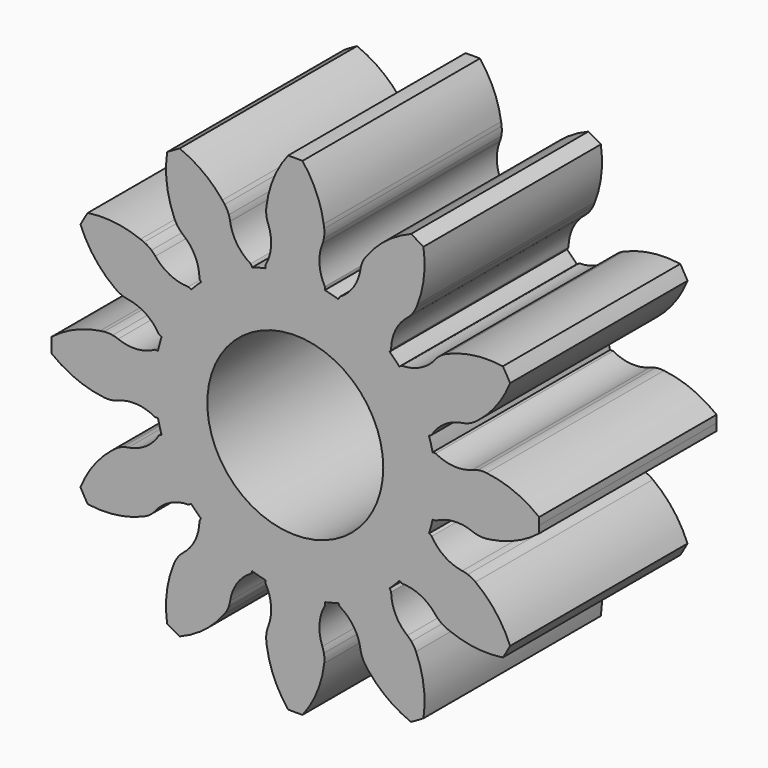
from build123d import *

# Parameters (mm, degrees)
F0_R     = 5.95
F1_DEPTH = 15


with BuildPart() as f1:
    # F0 (on Front) → F1 (new body)
    with BuildSketch(Plane.XZ):
        with BuildLine():
            ThreePointArc((16.4927779447, -0.4881348847), (16.4981943874, -0.2440941538), (16.5, 0))
            ThreePointArc((16.5, 0), (16.4981943874, 0.2440941538), (16.4927779447, 0.4881348847))
            ThreePointArc((16.4927779448, 0.4881348847), (14.8199031267, 1.4716268374), (12.9411319368, 1.9574101163))
            ThreePointArc((12.9411319368, 1.9574101163), (12.6443205895, 1.9691300904), (12.3490470013, 1.936759706))
            ThreePointArc((12.3490470013, 1.936759706), (12.4622046107, 0.9713167566), (12.5, 0))
            ThreePointArc((12.5, 0), (12.4622046107, -0.9713167566), (12.3490470013, -1.936759706))
            ThreePointArc((12.3490470013, -1.936759706), (12.6443205895, -1.9691300904), (12.9411319368, -1.9574101163))
            ThreePointArc((12.9411319368, -1.9574101163), (13.0706718945, -1.9413788034), (13.1998899951, -1.9229319577))
            ThreePointArc((13.1998899951, -1.9229319577), (14.9400467825, -1.4206061985), (16.4927779447, -0.4881348847))
        make_face()
        with BuildLine():
            ThreePointArc((12.3929060418, 4.9346370725), (13.6487631466, 6.2397423346), (14.5272321215, 7.8236517617))
            ThreePointArc((14.5272321215, 7.8236517617), (14.2894191624, 8.25), (14.0390972368, 8.669126183))
            ThreePointArc((14.0390972368, 8.669126183), (12.0985991706, 8.6844177894), (10.2286439528, 8.1657328548))
            ThreePointArc((10.2286439528, 8.1657328548), (9.9657377989, 8.0274769764), (9.7262085627, 7.8518066071))
            ThreePointArc((9.7262085627, 7.8518066071), (10.8253175473, 6.25), (11.6629682687, 4.4972403942))
            ThreePointArc((11.6629682687, 4.4972403942), (11.9348678893, 4.6168436131), (12.1860540692, 4.775399082))
            ThreePointArc((12.1860540692, 4.775399082), (12.2902233069, 4.8540525851), (12.3929060418, 4.9346370725))
        make_face()
        with BuildLine():
            ThreePointArc((14.0390972368, -8.669126183), (14.2894191624, -8.25), (14.5272321215, -7.8236517617))
            ThreePointArc((14.5272321215, -7.8236517617), (13.570226008, -6.1354853373), (12.1860540692, -4.775399082))
            ThreePointArc((12.1860540692, -4.775399082), (11.9348678893, -4.6168436131), (11.6629682687, -4.4972403942))
            ThreePointArc((11.6629682687, -4.4972403942), (10.8253175473, -6.25), (9.7262085627, -7.8518066071))
            ThreePointArc((9.7262085627, -7.8518066071), (9.9657377989, -8.0274769764), (10.2286439528, -8.1657328548))
            ThreePointArc((10.2286439528, -8.1657328548), (10.3488445035, -8.2166193094), (10.4699740841, -8.2652529226))
            ThreePointArc((10.4699740841, -8.2652529226), (12.2281569481, -8.7003044479), (14.0390972368, -8.669126183))
        make_face()
        with BuildLine():
            ThreePointArc((12.5, 0), (12.4622046107, 0.9713167566), (12.3490470013, 1.936759706))
            ThreePointArc((12.3490470013, 1.936759706), (12.163920368, 1.8932016239), (11.9837680157, 1.8322565103))
            ThreePointArc((11.9837680157, 1.8322565103), (10.7230754287, 1.6376307269), (9.5, 2))
            ThreePointArc((9.5, 2), (9.3935439053, 2.0073586069), (9.2870878105, 2))
            ThreePointArc((9.2870878105, 2), (9.4466219941, 1.0056504861), (9.5, 0))
            ThreePointArc((9.5, 0), (9.4466219941, -1.0056504861), (9.2870878105, -2))
            ThreePointArc((9.2870878105, -2), (9.3935439053, -2.0073586069), (9.5, -2))
            ThreePointArc((9.5, -2), (10.7230754287, -1.6376307269), (11.9837680157, -1.8322565103))
            ThreePointArc((11.9837680157, -1.8322565103), (12.163920368, -1.8932016239), (12.3490470013, -1.936759706))
            ThreePointArc((12.3490470013, -1.936759706), (12.4622046107, -0.9713167566), (12.5, 0))
        make_face()
        with BuildLine():
            ThreePointArc((8.2652529226, 10.4699740841), (8.7003044479, 12.2281569481), (8.669126183, 14.0390972368))
            ThreePointArc((8.669126183, 14.0390972368), (8.25, 14.2894191624), (7.8236517617, 14.5272321215))
            ThreePointArc((7.8236517617, 14.5272321215), (6.1354853373, 13.570226008), (4.775399082, 12.1860540692))
            ThreePointArc((4.775399082, 12.1860540692), (4.6168436131, 11.9348678893), (4.4972403942, 11.6629682687))
            ThreePointArc((4.4972403942, 11.6629682687), (6.25, 10.8253175473), (7.8518066071, 9.7262085627))
            ThreePointArc((7.8518066071, 9.7262085627), (8.0274769764, 9.9657377989), (8.1657328548, 10.2286439528))
            ThreePointArc((8.1657328548, 10.2286439528), (8.2166193094, 10.3488445035), (8.2652529226, 10.4699740841))
        make_face()
        with BuildLine():
            ThreePointArc((7.8236517617, -14.5272321215), (8.25, -14.2894191624), (8.669126183, -14.0390972368))
            ThreePointArc((8.669126183, -14.0390972368), (8.6844177894, -12.0985991706), (8.1657328548, -10.2286439528))
            ThreePointArc((8.1657328548, -10.2286439528), (8.0274769764, -9.9657377989), (7.8518066071, -9.7262085627))
            ThreePointArc((7.8518066071, -9.7262085627), (6.25, -10.8253175473), (4.4972403942, -11.6629682687))
            ThreePointArc((4.4972403942, -11.6629682687), (4.6168436131, -11.9348678893), (4.775399082, -12.1860540692))
            ThreePointArc((4.775399082, -12.1860540692), (4.8540525851, -12.2902233069), (4.9346370725, -12.3929060418))
            ThreePointArc((4.9346370725, -12.3929060418), (6.2397423346, -13.6487631466), (7.8236517617, -14.5272321215))
        make_face()
        with BuildLine():
            ThreePointArc((9.7262085627, -7.8518066071), (10.8253175473, -6.25), (11.6629682687, -4.4972403942))
            ThreePointArc((11.6629682687, -4.4972403942), (11.4808648602, -4.4423994832), (11.2943757898, -4.4051033237))
            ThreePointArc((11.2943757898, -4.4051033237), (10.1052710914, -3.9433079029), (9.227241336, -3.0179491924))
            ThreePointArc((9.227241336, -3.0179491924), (9.138726957, -2.9583484045), (9.0428539711, -2.9114930977))
            ThreePointArc((9.0428539711, -2.9114930977), (8.227241336, -4.75), (7.0428539711, -6.3755947128))
            ThreePointArc((7.0428539711, -6.3755947128), (7.13136835, -6.4351955007), (7.227241336, -6.4820508076))
            ThreePointArc((7.227241336, -6.4820508076), (8.4676403645, -6.7797675259), (9.4621192795, -7.578664692))
            ThreePointArc((9.4621192795, -7.578664692), (9.5876632363, -7.7215208848), (9.7262085627, -7.8518066071))
        make_face()
        with BuildLine():
            ThreePointArc((11.6629682687, 4.4972403942), (10.8253175473, 6.25), (9.7262085627, 7.8518066071))
            ThreePointArc((9.7262085627, 7.8518066071), (9.5876632363, 7.7215208848), (9.4621192795, 7.578664692))
            ThreePointArc((9.4621192795, 7.578664692), (8.4676403645, 6.7797675259), (7.227241336, 6.4820508076))
            ThreePointArc((7.227241336, 6.4820508076), (7.13136835, 6.4351955007), (7.0428539711, 6.3755947128))
            ThreePointArc((7.0428539711, 6.3755947128), (8.227241336, 4.75), (9.0428539711, 2.9114930977))
            ThreePointArc((9.0428539711, 2.9114930977), (9.138726957, 2.9583484045), (9.227241336, 3.0179491924))
            ThreePointArc((9.227241336, 3.0179491924), (10.1052710914, 3.9433079029), (11.2943757898, 4.4051033237))
            ThreePointArc((11.2943757898, 4.4051033237), (11.4808648602, 4.4423994832), (11.6629682687, 4.4972403942))
        make_face()
        with BuildLine():
            ThreePointArc((9.5, 0), (9.4466219941, 1.0056504861), (9.2870878105, 2))
            ThreePointArc((9.2870878105, 2), (9.1762953497, 2.4587809285), (9.0428539711, 2.9114930977))
            ThreePointArc((9.0428539711, 2.9114930977), (8.227241336, 4.75), (7.0428539711, 6.3755947128))
            ThreePointArc((7.0428539711, 6.3755947128), (6.7175144213, 6.7175144213), (6.3755947128, 7.0428539711))
            ThreePointArc((6.3755947128, 7.0428539711), (4.75, 8.227241336), (2.9114930977, 9.0428539711))
            ThreePointArc((2.9114930977, 9.0428539711), (2.4587809285, 9.1762953497), (2, 9.2870878105))
            ThreePointArc((2, 9.2870878105), (0, 9.5), (-2, 9.2870878105))
            ThreePointArc((-2, 9.2870878105), (-2.4587809285, 9.1762953497), (-2.9114930977, 9.0428539711))
            ThreePointArc((-2.9114930977, 9.0428539711), (-4.75, 8.227241336), (-6.3755947128, 7.0428539711))
            ThreePointArc((-6.3755947128, 7.0428539711), (-6.7175144213, 6.7175144213), (-7.0428539711, 6.3755947128))
            ThreePointArc((-7.0428539711, 6.3755947128), (-8.227241336, 4.75), (-9.0428539711, 2.9114930977))
            ThreePointArc((-9.0428539711, 2.9114930977), (-9.1762953497, 2.4587809285), (-9.2870878105, 2))
            ThreePointArc((-9.2870878105, 2), (-9.5, 0), (-9.2870878105, -2))
            ThreePointArc((-9.2870878105, -2), (-9.1762953497, -2.4587809285), (-9.0428539711, -2.9114930977))
            ThreePointArc((-9.0428539711, -2.9114930977), (-8.227241336, -4.75), (-7.0428539711, -6.3755947128))
            ThreePointArc((-7.0428539711, -6.3755947128), (-6.7175144213, -6.7175144213), (-6.3755947128, -7.0428539711))
            ThreePointArc((-6.3755947128, -7.0428539711), (-4.75, -8.227241336), (-2.9114930977, -9.0428539711))
            ThreePointArc((-2.9114930977, -9.0428539711), (-2.4587809285, -9.1762953497), (-2, -9.2870878105))
            ThreePointArc((-2, -9.2870878105), (0, -9.5), (2, -9.2870878105))
            ThreePointArc((2, -9.2870878105), (2.4587809285, -9.1762953497), (2.9114930977, -9.0428539711))
            ThreePointArc((2.9114930977, -9.0428539711), (4.75, -8.227241336), (6.3755947128, -7.0428539711))
            ThreePointArc((6.3755947128, -7.0428539711), (6.7175144213, -6.7175144213), (7.0428539711, -6.3755947128))
            ThreePointArc((7.0428539711, -6.3755947128), (8.227241336, -4.75), (9.0428539711, -2.9114930977))
            ThreePointArc((9.0428539711, -2.9114930977), (9.1762953497, -2.4587809285), (9.2870878105, -2))
            ThreePointArc((9.2870878105, -2), (9.4466219941, -1.0056504861), (9.5, 0))
        make_face()
        Circle(F0_R, mode=Mode.SUBTRACT)
        with BuildLine():
            ThreePointArc((-0.4881348847, -16.4927779447), (0, -16.5), (0.4881348847, -16.4927779447))
            ThreePointArc((0.4881348847, -16.4927779448), (1.4716268374, -14.8199031267), (1.9574101163, -12.9411319368))
            ThreePointArc((1.9574101163, -12.9411319368), (1.9691300904, -12.6443205895), (1.936759706, -12.3490470013))
            ThreePointArc((1.936759706, -12.3490470013), (0, -12.5), (-1.936759706, -12.3490470013))
            ThreePointArc((-1.936759706, -12.3490470013), (-1.9691300904, -12.6443205895), (-1.9574101163, -12.9411319368))
            ThreePointArc((-1.9574101163, -12.9411319368), (-1.9413788034, -13.0706718945), (-1.9229319577, -13.1998899951))
            ThreePointArc((-1.9229319577, -13.1998899951), (-1.4206061985, -14.9400467825), (-0.4881348847, -16.4927779447))
        make_face()
        with BuildLine():
            ThreePointArc((4.4972403942, -11.6629682687), (6.25, -10.8253175473), (7.8518066071, -9.7262085627))
            ThreePointArc((7.8518066071, -9.7262085627), (7.7215208848, -9.5876632363), (7.578664692, -9.4621192795))
            ThreePointArc((7.578664692, -9.4621192795), (6.7797675259, -8.4676403645), (6.4820508076, -7.227241336))
            ThreePointArc((6.4820508076, -7.227241336), (6.4351955007, -7.13136835), (6.3755947128, -7.0428539711))
            ThreePointArc((6.3755947128, -7.0428539711), (4.75, -8.227241336), (2.9114930977, -9.0428539711))
            ThreePointArc((2.9114930977, -9.0428539711), (2.9583484045, -9.138726957), (3.0179491924, -9.227241336))
            ThreePointArc((3.0179491924, -9.227241336), (3.9433079029, -10.1052710914), (4.4051033237, -11.2943757898))
            ThreePointArc((4.4051033237, -11.2943757898), (4.4423994832, -11.4808648602), (4.4972403942, -11.6629682687))
        make_face()
        with BuildLine():
            ThreePointArc((7.8518066071, 9.7262085627), (6.25, 10.8253175473), (4.4972403942, 11.6629682687))
            ThreePointArc((4.4972403942, 11.6629682687), (4.4423994832, 11.4808648602), (4.4051033237, 11.2943757898))
            ThreePointArc((4.4051033237, 11.2943757898), (3.9433079029, 10.1052710914), (3.0179491924, 9.227241336))
            ThreePointArc((3.0179491924, 9.227241336), (2.9583484045, 9.138726957), (2.9114930977, 9.0428539711))
            ThreePointArc((2.9114930977, 9.0428539711), (4.75, 8.227241336), (6.3755947128, 7.0428539711))
            ThreePointArc((6.3755947128, 7.0428539711), (6.4351955007, 7.13136835), (6.4820508076, 7.227241336))
            ThreePointArc((6.4820508076, 7.227241336), (6.7797675259, 8.4676403645), (7.578664692, 9.4621192795))
            ThreePointArc((7.578664692, 9.4621192795), (7.7215208848, 9.5876632363), (7.8518066071, 9.7262085627))
        make_face()
        with BuildLine():
            ThreePointArc((1.9229319577, 13.1998899951), (1.4206061985, 14.9400467825), (0.4881348847, 16.4927779447))
            ThreePointArc((0.4881348847, 16.4927779447), (0, 16.5), (-0.4881348847, 16.4927779447))
            ThreePointArc((-0.4881348847, 16.4927779448), (-1.4716268374, 14.8199031267), (-1.9574101163, 12.9411319368))
            ThreePointArc((-1.9574101163, 12.9411319368), (-1.9691300904, 12.6443205895), (-1.936759706, 12.3490470013))
            ThreePointArc((-1.936759706, 12.3490470013), (-0.9713167566, 12.4622046107), (0, 12.5))
            Line((0, 12.5), (1.9229319577, 13.1998899951))
        make_face()
        with BuildLine():
            ThreePointArc((-8.669126183, -14.0390972368), (-8.25, -14.2894191624), (-7.8236517617, -14.5272321215))
            ThreePointArc((-7.8236517617, -14.5272321215), (-6.1354853373, -13.570226008), (-4.775399082, -12.1860540692))
            ThreePointArc((-4.775399082, -12.1860540692), (-4.6168436131, -11.9348678893), (-4.4972403942, -11.6629682687))
            ThreePointArc((-4.4972403942, -11.6629682687), (-6.25, -10.8253175473), (-7.8518066071, -9.7262085627))
            ThreePointArc((-7.8518066071, -9.7262085627), (-8.0274769764, -9.9657377989), (-8.1657328548, -10.2286439528))
            ThreePointArc((-8.1657328548, -10.2286439528), (-8.2166193094, -10.3488445035), (-8.2652529226, -10.4699740841))
            ThreePointArc((-8.2652529226, -10.4699740841), (-8.7003044479, -12.2281569481), (-8.669126183, -14.0390972368))
        make_face()
        with BuildLine():
            ThreePointArc((-1.936759706, -12.3490470013), (0, -12.5), (1.936759706, -12.3490470013))
            ThreePointArc((1.936759706, -12.3490470013), (1.8932016239, -12.163920368), (1.8322565103, -11.9837680157))
            ThreePointArc((1.8322565103, -11.9837680157), (1.6376307269, -10.7230754287), (2, -9.5))
            ThreePointArc((2, -9.5), (2.0073586069, -9.3935439053), (2, -9.2870878105))
            ThreePointArc((2, -9.2870878105), (0, -9.5), (-2, -9.2870878105))
            ThreePointArc((-2, -9.2870878105), (-2.0073586069, -9.3935439053), (-2, -9.5))
            ThreePointArc((-2, -9.5), (-1.6376307269, -10.7230754287), (-1.8322565103, -11.9837680157))
            ThreePointArc((-1.8322565103, -11.9837680157), (-1.8932016239, -12.163920368), (-1.936759706, -12.3490470013))
        make_face()
        with BuildLine():
            ThreePointArc((1.9574101163, 12.9411319368), (1.9413788034, 13.0706718945), (1.9229319577, 13.1998899951))
            Line((1.9229319577, 13.1998899951), (0, 12.5))
            ThreePointArc((0, 12.5), (0.9713167566, 12.4622046107), (1.936759706, 12.3490470013))
            ThreePointArc((1.936759706, 12.3490470013), (1.9691300904, 12.6443205895), (1.9574101163, 12.9411319368))
        make_face()
        with BuildLine():
            ThreePointArc((2, 9.2870878105), (2.0073586069, 9.3935439053), (2, 9.5))
            ThreePointArc((2, 9.5), (1.6376307269, 10.7230754287), (1.8322565103, 11.9837680157))
            ThreePointArc((1.8322565103, 11.9837680157), (1.8932016239, 12.163920368), (1.936759706, 12.3490470013))
            ThreePointArc((1.936759706, 12.3490470013), (0.9713167566, 12.4622046107), (0, 12.5))
            ThreePointArc((0, 12.5), (-0.9713167566, 12.4622046107), (-1.936759706, 12.3490470013))
            ThreePointArc((-1.936759706, 12.3490470013), (-1.8932016239, 12.163920368), (-1.8322565103, 11.9837680157))
            ThreePointArc((-1.8322565103, 11.9837680157), (-1.6376307269, 10.7230754287), (-2, 9.5))
            ThreePointArc((-2, 9.5), (-2.0073586069, 9.3935439053), (-2, 9.2870878105))
            ThreePointArc((-2, 9.2870878105), (0, 9.5), (2, 9.2870878105))
        make_face()
        with BuildLine():
            ThreePointArc((-14.5272321215, -7.8236517617), (-14.2894191624, -8.25), (-14.0390972368, -8.669126183))
            ThreePointArc((-14.0390972368, -8.669126183), (-12.0985991706, -8.6844177894), (-10.2286439528, -8.1657328548))
            ThreePointArc((-10.2286439528, -8.1657328548), (-9.9657377989, -8.0274769764), (-9.7262085627, -7.8518066071))
            ThreePointArc((-9.7262085627, -7.8518066071), (-10.8253175473, -6.25), (-11.6629682687, -4.4972403942))
            ThreePointArc((-11.6629682687, -4.4972403942), (-11.9348678893, -4.6168436131), (-12.1860540692, -4.775399082))
            ThreePointArc((-12.1860540692, -4.775399082), (-12.2902233069, -4.8540525851), (-12.3929060418, -4.9346370725))
            ThreePointArc((-12.3929060418, -4.9346370725), (-13.6487631466, -6.2397423346), (-14.5272321215, -7.8236517617))
        make_face()
        with BuildLine():
            ThreePointArc((-7.8518066071, -9.7262085627), (-6.25, -10.8253175473), (-4.4972403942, -11.6629682687))
            ThreePointArc((-4.4972403942, -11.6629682687), (-4.4423994832, -11.4808648602), (-4.4051033237, -11.2943757898))
            ThreePointArc((-4.4051033237, -11.2943757898), (-3.9433079029, -10.1052710914), (-3.0179491924, -9.227241336))
            ThreePointArc((-3.0179491924, -9.227241336), (-2.9583484045, -9.138726957), (-2.9114930977, -9.0428539711))
            ThreePointArc((-2.9114930977, -9.0428539711), (-4.75, -8.227241336), (-6.3755947128, -7.0428539711))
            ThreePointArc((-6.3755947128, -7.0428539711), (-6.4351955007, -7.13136835), (-6.4820508076, -7.227241336))
            ThreePointArc((-6.4820508076, -7.227241336), (-6.7797675259, -8.4676403645), (-7.578664692, -9.4621192795))
            ThreePointArc((-7.578664692, -9.4621192795), (-7.7215208848, -9.5876632363), (-7.8518066071, -9.7262085627))
        make_face()
        with BuildLine():
            ThreePointArc((-4.9346370725, 12.3929060418), (-6.2397423346, 13.6487631466), (-7.8236517617, 14.5272321215))
            ThreePointArc((-7.8236517617, 14.5272321215), (-8.25, 14.2894191624), (-8.669126183, 14.0390972368))
            ThreePointArc((-8.669126183, 14.0390972368), (-8.6844177894, 12.0985991706), (-8.1657328548, 10.2286439528))
            ThreePointArc((-8.1657328548, 10.2286439528), (-8.0274769764, 9.9657377989), (-7.8518066071, 9.7262085627))
            ThreePointArc((-7.8518066071, 9.7262085627), (-6.25, 10.8253175473), (-4.4972403942, 11.6629682687))
            ThreePointArc((-4.4972403942, 11.6629682687), (-4.6168436131, 11.9348678893), (-4.775399082, 12.1860540692))
            ThreePointArc((-4.775399082, 12.1860540692), (-4.8540525851, 12.2902233069), (-4.9346370725, 12.3929060418))
        make_face()
        with BuildLine():
            ThreePointArc((-6.3755947128, 7.0428539711), (-4.75, 8.227241336), (-2.9114930977, 9.0428539711))
            ThreePointArc((-2.9114930977, 9.0428539711), (-2.9583484045, 9.138726957), (-3.0179491924, 9.227241336))
            ThreePointArc((-3.0179491924, 9.227241336), (-3.9433079029, 10.1052710914), (-4.4051033237, 11.2943757898))
            ThreePointArc((-4.4051033237, 11.2943757898), (-4.4423994832, 11.4808648602), (-4.4972403942, 11.6629682687))
            ThreePointArc((-4.4972403942, 11.6629682687), (-6.25, 10.8253175473), (-7.8518066071, 9.7262085627))
            ThreePointArc((-7.8518066071, 9.7262085627), (-7.7215208848, 9.5876632363), (-7.578664692, 9.4621192795))
            ThreePointArc((-7.578664692, 9.4621192795), (-6.7797675259, 8.4676403645), (-6.4820508076, 7.227241336))
            ThreePointArc((-6.4820508076, 7.227241336), (-6.4351955007, 7.13136835), (-6.3755947128, 7.0428539711))
        make_face()
        with BuildLine():
            ThreePointArc((-16.4927779447, 0.4881348847), (-16.5, 0), (-16.4927779447, -0.4881348847))
            ThreePointArc((-16.4927779448, -0.4881348847), (-14.8199031267, -1.4716268374), (-12.9411319368, -1.9574101163))
            ThreePointArc((-12.9411319368, -1.9574101163), (-12.6443205895, -1.9691300904), (-12.3490470013, -1.936759706))
            ThreePointArc((-12.3490470013, -1.936759706), (-12.5, 0), (-12.3490470013, 1.936759706))
            ThreePointArc((-12.3490470013, 1.936759706), (-12.6443205895, 1.9691300904), (-12.9411319368, 1.9574101163))
            ThreePointArc((-12.9411319368, 1.9574101163), (-13.0706718945, 1.9413788034), (-13.1998899951, 1.9229319577))
            ThreePointArc((-13.1998899951, 1.9229319577), (-14.9400467825, 1.4206061985), (-16.4927779447, 0.4881348847))
        make_face()
        with BuildLine():
            ThreePointArc((-11.6629682687, -4.4972403942), (-10.8253175473, -6.25), (-9.7262085627, -7.8518066071))
            ThreePointArc((-9.7262085627, -7.8518066071), (-9.5876632363, -7.7215208848), (-9.4621192795, -7.578664692))
            ThreePointArc((-9.4621192795, -7.578664692), (-8.4676403645, -6.7797675259), (-7.227241336, -6.4820508076))
            ThreePointArc((-7.227241336, -6.4820508076), (-7.13136835, -6.4351955007), (-7.0428539711, -6.3755947128))
            ThreePointArc((-7.0428539711, -6.3755947128), (-8.227241336, -4.75), (-9.0428539711, -2.9114930977))
            ThreePointArc((-9.0428539711, -2.9114930977), (-9.138726957, -2.9583484045), (-9.227241336, -3.0179491924))
            ThreePointArc((-9.227241336, -3.0179491924), (-10.1052710914, -3.9433079029), (-11.2943757898, -4.4051033237))
            ThreePointArc((-11.2943757898, -4.4051033237), (-11.4808648602, -4.4423994832), (-11.6629682687, -4.4972403942))
        make_face()
        with BuildLine():
            ThreePointArc((-10.4699740841, 8.2652529226), (-12.2281569481, 8.7003044479), (-14.0390972368, 8.669126183))
            ThreePointArc((-14.0390972368, 8.669126183), (-14.2894191624, 8.25), (-14.5272321215, 7.8236517617))
            ThreePointArc((-14.5272321215, 7.8236517617), (-13.570226008, 6.1354853373), (-12.1860540692, 4.775399082))
            ThreePointArc((-12.1860540692, 4.775399082), (-11.9348678893, 4.6168436131), (-11.6629682687, 4.4972403942))
            ThreePointArc((-11.6629682687, 4.4972403942), (-10.8253175473, 6.25), (-9.7262085627, 7.8518066071))
            ThreePointArc((-9.7262085627, 7.8518066071), (-9.9657377989, 8.0274769764), (-10.2286439528, 8.1657328548))
            ThreePointArc((-10.2286439528, 8.1657328548), (-10.3488445035, 8.2166193094), (-10.4699740841, 8.2652529226))
        make_face()
        with BuildLine():
            ThreePointArc((-9.0428539711, 2.9114930977), (-8.227241336, 4.75), (-7.0428539711, 6.3755947128))
            ThreePointArc((-7.0428539711, 6.3755947128), (-7.13136835, 6.4351955007), (-7.227241336, 6.4820508076))
            ThreePointArc((-7.227241336, 6.4820508076), (-8.4676403645, 6.7797675259), (-9.4621192795, 7.578664692))
            ThreePointArc((-9.4621192795, 7.578664692), (-9.5876632363, 7.7215208848), (-9.7262085627, 7.8518066071))
            ThreePointArc((-9.7262085627, 7.8518066071), (-10.8253175473, 6.25), (-11.6629682687, 4.4972403942))
            ThreePointArc((-11.6629682687, 4.4972403942), (-11.4808648602, 4.4423994832), (-11.2943757898, 4.4051033237))
            ThreePointArc((-11.2943757898, 4.4051033237), (-10.1052710914, 3.9433079029), (-9.227241336, 3.0179491924))
            ThreePointArc((-9.227241336, 3.0179491924), (-9.138726957, 2.9583484045), (-9.0428539711, 2.9114930977))
        make_face()
        with BuildLine():
            ThreePointArc((-12.3490470013, 1.936759706), (-12.5, 0), (-12.3490470013, -1.936759706))
            ThreePointArc((-12.3490470013, -1.936759706), (-12.163920368, -1.8932016239), (-11.9837680157, -1.8322565103))
            ThreePointArc((-11.9837680157, -1.8322565103), (-10.7230754287, -1.6376307269), (-9.5, -2))
            ThreePointArc((-9.5, -2), (-9.3935439053, -2.0073586069), (-9.2870878105, -2))
            ThreePointArc((-9.2870878105, -2), (-9.5, 0), (-9.2870878105, 2))
            ThreePointArc((-9.2870878105, 2), (-9.3935439053, 2.0073586069), (-9.5, 2))
            ThreePointArc((-9.5, 2), (-10.7230754287, 1.6376307269), (-11.9837680157, 1.8322565103))
            ThreePointArc((-11.9837680157, 1.8322565103), (-12.163920368, 1.8932016239), (-12.3490470013, 1.936759706))
        make_face()
    extrude(amount=F1_DEPTH)


solid = f1.part
